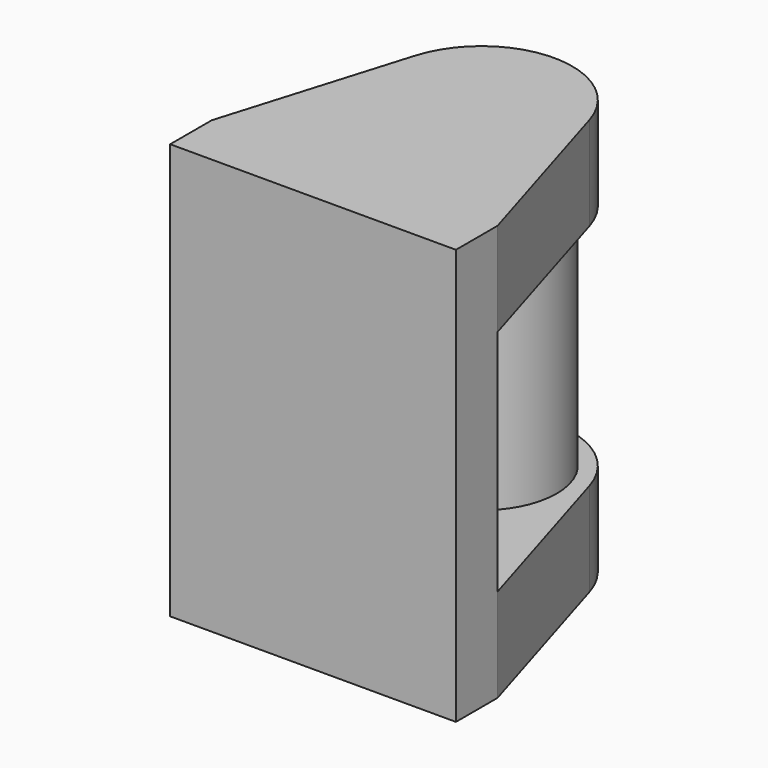
from build123d import *

# Parameters (mm, degrees)
F0_W     = 2.75
F0_H     = 1
F0_R     = 1.45
F1_DEPTH = 1.8
F2_DEPTH = 4


# Not quite as in the source:
# - a feature of the source that left no trace in its solid (it failed there, or was rolled back) is left out


with BuildPart() as f1:
    # F0 (on Top) → F1 (new body)
    with BuildSketch(Plane.XY):
        with Locations((1.375, 0.5)):
            Rectangle(F0_W, F0_H)
        with Locations((-1.375, 0.5)):
            Rectangle(F0_W, F0_H)
        with BuildLine():
            Line((0, 2.3), (0, 1))
            Line((0, 1), (2.75, 1))
            Line((2.75, 1), (1.675161779, 4.5562934073))
            ThreePointArc((1.675161779, 4.5562934073), (1.7311893474, 4.3058973298), (1.75, 4.05))
            ThreePointArc((1.75, 4.05), (1.2374368671, 2.8125631329), (0, 2.3))
        make_face()
        with BuildLine():
            Line((-2.75, 1), (0, 1))
            Line((0, 1), (0, 2.3))
            ThreePointArc((0, 2.3), (-1.4050824643, 3.0068110101), (-1.675161779, 4.5562934073))
            Line((-1.675161779, 4.5562934073), (-2.75, 1))
        make_face()
        with BuildLine():
            ThreePointArc((-1.675161779, 4.5562934073), (-1.4050824643, 3.0068110101), (0, 2.3))
            ThreePointArc((0, 2.3), (1.2374368671, 2.8125631329), (1.75, 4.05))
            ThreePointArc((1.75, 4.05), (1.7311893474, 4.3058973298), (1.675161779, 4.5562934073))
            ThreePointArc((1.675161779, 4.5562934073), (0, 5.8), (-1.675161779, 4.5562934073))
        make_face()
        with Locations((0, 4.05)):
            Circle(F0_R, mode=Mode.SUBTRACT)
        with Locations((0, 4.05)):
            Circle(F0_R)
    extrude(amount=F1_DEPTH)

    # F0 (on Top) → F2 (join)
    with BuildSketch(Plane.XY):
        with Locations((0, 4.05)):
            Circle(F0_R)
        with Locations((-1.375, 0.5)):
            Rectangle(F0_W, F0_H)
        with Locations((1.375, 0.5)):
            Rectangle(F0_W, F0_H)
    extrude(amount=F2_DEPTH)

    # F4: F1 across plane


with BuildPart() as f1_1:
    add(f1.part)
    add(f1.part.mirror(Plane.XY.offset(4)))


solid = f1_1.part
